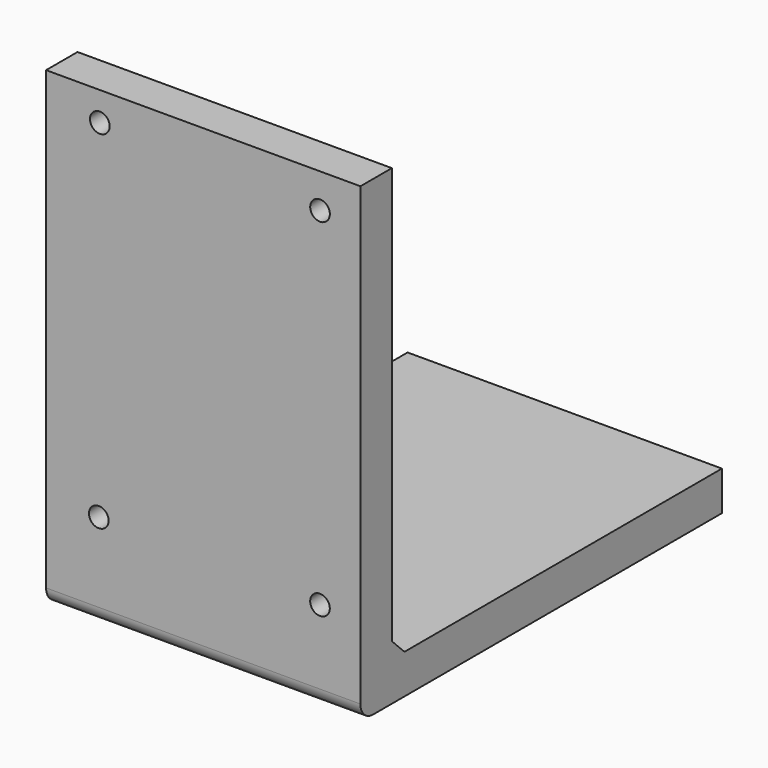
from build123d import *

# Parameters (mm, degrees)
F0_W     = 101.6
F0_H     = 152.4
F1_DEPTH = 6.35
F2_W     = 139.7
F2_H     = 76.2
F3_DEPTH = 50.8
F4_DEPTH = 63.5
F5_SIZE  = 5.08
F6_R     = 5.08
F7_R     = 3.175
F8_DEPTH = 12.7


with BuildPart() as f1:
    # F0 (on Front) → F1 (new body, symmetric)
    with BuildSketch(Plane.XZ):
        Rectangle(F0_W, F0_H)
    extrude(amount=F1_DEPTH, both=True)

    # F2 (on Right) → F3 (join, symmetric)
    with BuildSketch(Plane.YZ):
        with Locations((69.85, -38.1)):
            Rectangle(F2_W, F2_H)
    extrude(amount=F3_DEPTH, both=True)

    # F4 (cut): a face of the model
    f4_faces = [f1.faces().sort_by_distance(p)[0] for p in [
        (0, 73.025, 0),
    ]]
    extrude(f4_faces, amount=-F4_DEPTH, mode=Mode.SUBTRACT)

    # F5
    f5_edges = [f1.edges().sort_by_distance(p)[0] for p in [
        (0, 6.35, -63.5),
    ]]
    chamfer(f5_edges, length=F5_SIZE)

    # F6
    f6_edges = [f1.edges().sort_by_distance(p)[0] for p in [
        (0, -6.35, -76.2),
    ]]
    fillet(f6_edges, radius=F6_R)

    # F7 (on face) → F8 (cut)
    with BuildSketch(Plane(origin=(0, 6.35, 0), x_dir=(-1, 0, 0), z_dir=(0, 1, 0))):
        with Locations((-37.7415953271, 65.0431930406)):
            Circle(F7_R)
        with Locations((33.4293011874, 66.8958395785)):
            Circle(F7_R)
        with Locations((33.7640900696, -45.4423770942)):
            Circle(F7_R)
        with Locations((-37.7306027449, -47.1545040206)):
            Circle(F7_R)
    extrude(amount=-F8_DEPTH, mode=Mode.SUBTRACT)


solid = f1.part
